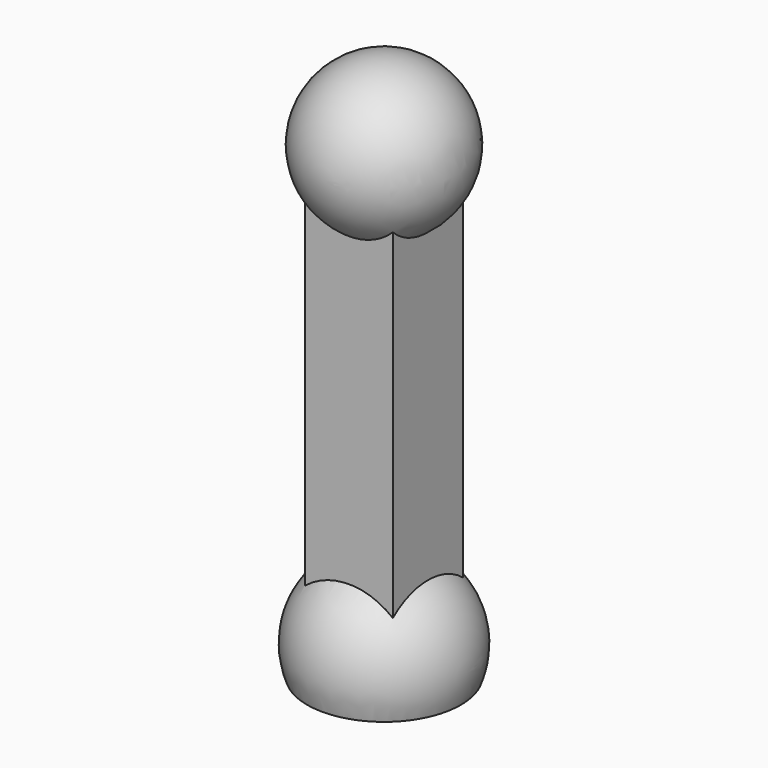
from build123d import *
from build123d import SkipClean  # not in build123d's __all__

# Parameters (mm, degrees)
F2_W     = 8
F2_H     = 8
F3_DEPTH = 40
F4_R     = 7
F5_DEPTH = 7.5
F6_W     = 4
F6_H     = 8
F8_W     = 4
F8_H     = 8


# Not quite as in the source:
# - a feature names something its author has since deleted; it is built from what else it names


with BuildPart() as f1:
    # F0 (on Top) → F1 (revolve)
    with BuildSketch(Plane.XY):
        with BuildLine():
            Line((7, 0), (7.5, 0))
            ThreePointArc((7.5, 0), (0, 7.5), (-7.5, 0))
            Line((-7.5, 0), (-7, 0))
            ThreePointArc((-7, 0), (0, 7), (7, 0))
        make_face()
    revolve(axis=Axis((0, 0, 0), (-1, 0, 0)))

    # F2 (on Top) → F3 (join)
    with BuildSketch(Plane.XY):
        Rectangle(F2_W, F2_H)
    extrude(amount=F3_DEPTH)

    # F4 (on Top) → F5 (cut)
    with BuildSketch(Plane.XY):
        Circle(F4_R)
    extrude(amount=-F5_DEPTH, mode=Mode.SUBTRACT)

    # F6 (on face) → F7 (revolve, cut)
    with BuildSketch(Plane(origin=(0, 0, 0), x_dir=(1, 0, 0), z_dir=(0, 0, -1))):
        with BuildLine():
            ThreePointArc((0, -7), (7, 0), (0, 7))
            Line((0, 7), (0, 4))
            Line((0, 4), (4, 4))
            Line((4, 4), (4, -4))
            Line((4, -4), (0, -4))
            Line((0, -4), (0, -7))
        make_face()
        with Locations((2, 0)):
            Rectangle(F6_W, F6_H)
    with SkipClean():  # cleaning this boolean's faces spoils the solid; the shape is the same uncleaned
        revolve(axis=Axis((0, 0, 0), (0, 1, 0)), mode=Mode.SUBTRACT)

    # F8 (on face) → F9 (revolve)
    with BuildSketch(Plane.XY.offset(40)):
        with BuildLine():
            ThreePointArc((0, -7), (7, 0), (0, 7))
            Line((0, 7), (0, 4))
            Line((0, 4), (4, 4))
            Line((4, 4), (4, -4))
            Line((4, -4), (0, -4))
            Line((0, -4), (0, -7))
        make_face()
        with Locations((2, 0)):
            Rectangle(F8_W, F8_H)
    with SkipClean():  # cleaning this boolean's faces spoils the solid; the shape is the same uncleaned
        revolve(axis=Axis((0, 0, 40), (0, -1, 0)))


solid = f1.part
